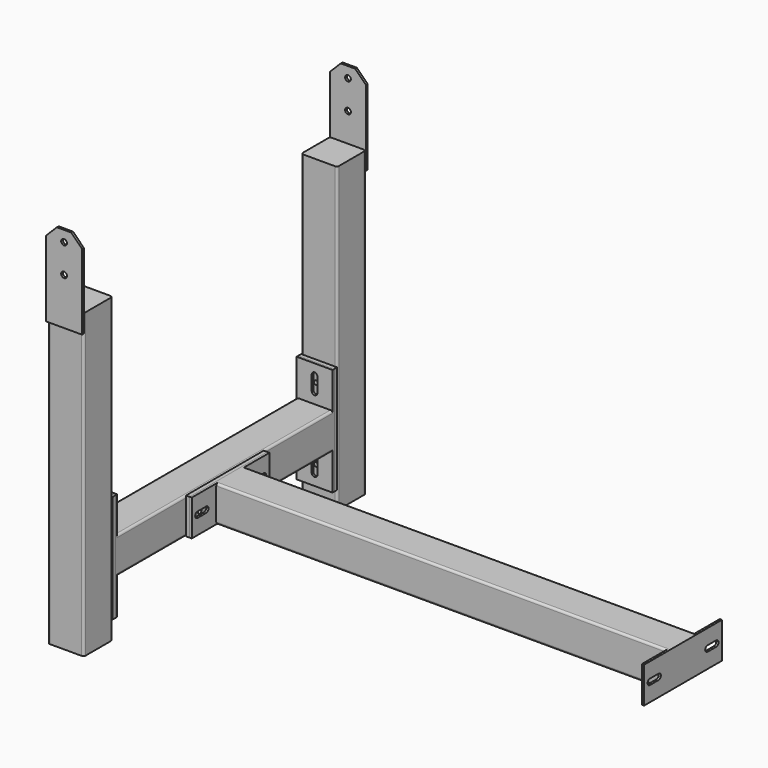
from build123d import *

# Parameters (mm, degrees)
F1_DEPTH  = 420
F2_W      = 50
F2_H      = 150
F2_R      = 3
F3_DEPTH  = 5
F5_DEPTH  = 1.5
F6_W      = 50
F6_H      = 120
F6_R      = 4
F7_DEPTH  = 3
F8_SIZE   = 15
F11_W     = 50
F11_H     = 150
F12_DEPTH = 3
F15_DEPTH = 374
F17_W     = 135
F17_H     = 50
F17_R     = 3
F18_DEPTH = 5
F19_W     = 135
F19_H     = 50
F19_R     = 4
F20_DEPTH = 3
F23_DEPTH = 625.5
F25_DEPTH = 3.001


# Not quite as in the source:
# - a pattern or mirror of a feature is missing from the dataset's text; its kind, count and spacing are read off the source's solid


with BuildPart() as f1:
    # F0 (on Top) → F1 (new body)
    with BuildSketch(Plane.XY):
        with BuildLine():
            Line((-22, -25), (22, -25))
            ThreePointArc((22, -25), (24.1213203436, -24.1213203436), (25, -22))
            Line((25, -22), (25, 22))
            ThreePointArc((25, 22), (24.1213203436, 24.1213203436), (22, 25))
            Line((22, 25), (-22, 25))
            ThreePointArc((-22, 25), (-24.1213203436, 24.1213203436), (-25, 22))
            Line((-25, 22), (-25, -22))
            ThreePointArc((-25, -22), (-24.1213203436, -24.1213203436), (-22, -25))
        make_face()
        with BuildLine():
            ThreePointArc((22, 23.5), (23.0606601718, 23.0606601718), (23.5, 22))
            Line((23.5, 22), (23.5, -22))
            ThreePointArc((23.5, -22), (23.0606601718, -23.0606601718), (22, -23.5))
            Line((22, -23.5), (-22, -23.5))
            ThreePointArc((-22, -23.5), (-23.0606601718, -23.0606601718), (-23.5, -22))
            Line((-23.5, -22), (-23.5, 22))
            ThreePointArc((-23.5, 22), (-23.0606601718, 23.0606601718), (-22, 23.5))
            Line((-22, 23.5), (22, 23.5))
        make_face(mode=Mode.SUBTRACT)
    extrude(amount=F1_DEPTH)

    # F2 (on face) → F3 (join)
    with BuildSketch(Plane(origin=(0, 25, 0), x_dir=(-1, 0, 0), z_dir=(0, 1, 0))):
        with Locations((0, 100)):
            Rectangle(F2_W, F2_H)
        with Locations((0, 50)):
            Circle(F2_R, mode=Mode.SUBTRACT)
        with Locations((0, 150)):
            Circle(F2_R, mode=Mode.SUBTRACT)
    extrude(amount=F3_DEPTH)

    # F4 (on face) → F5 (join)
    with BuildSketch(Plane.XY.offset(420)):
        with BuildLine():
            ThreePointArc((23.5, 22), (23.0606601718, 23.0606601718), (22, 23.5))
            Line((22, 23.5), (-22, 23.5))
            ThreePointArc((-22, 23.5), (-23.0606601718, 23.0606601718), (-23.5, 22))
            Line((-23.5, 22), (-23.5, -22))
            ThreePointArc((-23.5, -22), (-23.0606601718, -23.0606601718), (-22, -23.5))
            Line((-22, -23.5), (22, -23.5))
            ThreePointArc((22, -23.5), (23.0606601718, -23.0606601718), (23.5, -22))
            Line((23.5, -22), (23.5, 22))
        make_face()
    extrude(amount=-F5_DEPTH)

    # F6 (on face) → F7 (join)
    with BuildSketch(Plane.XZ.offset(25)):
        with Locations((0, 455)):
            Rectangle(F6_W, F6_H)
        with Locations((0, 460)):
            Circle(F6_R, mode=Mode.SUBTRACT)
        with Locations((0, 500)):
            Circle(F6_R, mode=Mode.SUBTRACT)
    extrude(amount=F7_DEPTH)

    # F8
    f8_edges = [f1.edges().sort_by_distance(p)[0] for p in [
        (25, -26.5, 515),
        (-25, -26.5, 515),
    ]]
    chamfer(f8_edges, length=F8_SIZE)


with BuildPart() as f10_1:
    # F10: instance of F1
    add(f1.part.mirror(Plane(origin=(0, 220, 463.1674453561), x_dir=(1, 0, 0), z_dir=(0, 1, 0))))


with BuildPart() as f12:
    # F11 (on face) → F12 (new body)
    with BuildSketch(Plane(origin=(0, 30, 0), x_dir=(-1, 0, 0), z_dir=(0, 1, 0))):
        with Locations((0, 100)):
            Rectangle(F11_W, F11_H)
        with BuildLine():
            Line((-4, 40), (-4, 60))
            ThreePointArc((-4, 60), (0, 64), (4, 60))
            Line((4, 60), (4, 40))
            ThreePointArc((4, 40), (0, 36), (-4, 40))
        make_face(mode=Mode.SUBTRACT)
        with BuildLine():
            Line((4, 160), (4, 140))
            ThreePointArc((4, 140), (0, 136), (-4, 140))
            Line((-4, 140), (-4, 160))
            ThreePointArc((-4, 160), (0, 164), (4, 160))
        make_face(mode=Mode.SUBTRACT)
    extrude(amount=F12_DEPTH)


with BuildPart() as f13_1:
    # F13: instance of F12
    add(f12.part.mirror(Plane(origin=(0, 220, 463.1674453561), x_dir=(1, 0, 0), z_dir=(0, 1, 0))))


with BuildPart() as f12_1:
    add(f12.part)

    add(f13_1.part)  # F15 merges F13_1
    # F14 (on face) → F15 (join, through all)
    with BuildSketch(Plane(origin=(0, 33, 0), x_dir=(-1, 0, 0), z_dir=(0, 1, 0))):
        with BuildLine():
            Line((-22, 75), (22, 75))
            ThreePointArc((22, 75), (24.1213203436, 75.8786796564), (25, 78))
            Line((25, 78), (25, 122))
            ThreePointArc((25, 122), (24.1213203436, 124.1213203436), (22, 125))
            Line((22, 125), (-22, 125))
            ThreePointArc((-22, 125), (-24.1213203436, 124.1213203436), (-25, 122))
            Line((-25, 122), (-25, 78))
            ThreePointArc((-25, 78), (-24.1213203436, 75.8786796564), (-22, 75))
        make_face()
        with BuildLine():
            ThreePointArc((22, 123.5), (23.0606601718, 123.0606601718), (23.5, 122))
            Line((23.5, 122), (23.5, 78))
            ThreePointArc((23.5, 78), (23.0606601718, 76.9393398282), (22, 76.5))
            Line((22, 76.5), (-22, 76.5))
            ThreePointArc((-22, 76.5), (-23.0606601718, 76.9393398282), (-23.5, 78))
            Line((-23.5, 78), (-23.5, 122))
            ThreePointArc((-23.5, 122), (-23.0606601718, 123.0606601718), (-22, 123.5))
            Line((-22, 123.5), (22, 123.5))
        make_face(mode=Mode.SUBTRACT)
    extrude(amount=F15_DEPTH)

    # F17 (on face) → F18 (join)
    with BuildSketch(Plane.YZ.offset(25)):
        with Locations((220, 100)):
            Rectangle(F17_W, F17_H)
        with Locations((170, 100)):
            Circle(F17_R, mode=Mode.SUBTRACT)
        with Locations((270, 100)):
            Circle(F17_R, mode=Mode.SUBTRACT)
    extrude(amount=F18_DEPTH)


with BuildPart() as f20:
    # F19 (on face) → F20 (new body)
    with BuildSketch(Plane.YZ.offset(30)):
        with Locations((220, 100)):
            Rectangle(F19_W, F19_H)
        with Locations((170, 100)):
            Circle(F19_R, mode=Mode.SUBTRACT)
        with Locations((270, 100)):
            Circle(F19_R, mode=Mode.SUBTRACT)
    extrude(amount=F20_DEPTH)


with BuildPart() as f21_1:
    # F21: instance of F20
    add(f20.part.mirror(Plane(origin=(345.75, 0, 210), x_dir=(0, 1, 0), z_dir=(1, 0, 0))))


with BuildPart() as f20_1:
    add(f20.part)

    add(f21_1.part)  # F23 merges F21_1
    # F22 (on face) → F23 (join, through all)
    with BuildSketch(Plane.YZ.offset(33)):
        with BuildLine():
            Line((198, 75), (242, 75))
            ThreePointArc((242, 75), (244.1213203436, 75.8786796564), (245, 78))
            Line((245, 78), (245, 122))
            ThreePointArc((245, 122), (244.1213203436, 124.1213203436), (242, 125))
            Line((242, 125), (198, 125))
            ThreePointArc((198, 125), (195.8786796564, 124.1213203436), (195, 122))
            Line((195, 122), (195, 78))
            ThreePointArc((195, 78), (195.8786796564, 75.8786796564), (198, 75))
        make_face()
        with BuildLine():
            ThreePointArc((242, 123.5), (243.0606601718, 123.0606601718), (243.5, 122))
            Line((243.5, 122), (243.5, 78))
            ThreePointArc((243.5, 78), (243.0606601718, 76.9393398282), (242, 76.5))
            Line((242, 76.5), (198, 76.5))
            ThreePointArc((198, 76.5), (196.9393398282, 76.9393398282), (196.5, 78))
            Line((196.5, 78), (196.5, 122))
            ThreePointArc((196.5, 122), (196.9393398282, 123.0606601718), (198, 123.5))
            Line((198, 123.5), (242, 123.5))
        make_face(mode=Mode.SUBTRACT)
    extrude(amount=F23_DEPTH)

    # F24 (on face) → F25 (cut, through all)
    with BuildSketch(Plane.YZ.offset(661.5)):
        with BuildLine():
            Line((162.5, 96), (177.5, 96))
            ThreePointArc((177.5, 96), (181.5, 100), (177.5, 104))
            Line((177.5, 104), (162.5, 104))
            ThreePointArc((162.5, 104), (158.5, 100), (162.5, 96))
        make_face()
        with BuildLine():
            ThreePointArc((262.5, 104), (258.5, 100), (262.5, 96))
            Line((262.5, 96), (277.5, 96))
            ThreePointArc((277.5, 96), (281.5, 100), (277.5, 104))
            Line((277.5, 104), (262.5, 104))
        make_face()
    f25 = extrude(amount=-F25_DEPTH, mode=Mode.SUBTRACT)

    # F25_copies: F25 across plane
    add(f25.mirror(Plane(origin=(345.75, 0, 0), x_dir=(0, 0, -1), z_dir=(-1, 0, 0))), mode=Mode.SUBTRACT)


solid = Compound([f1.part, f10_1.part, f12_1.part, f20_1.part])
